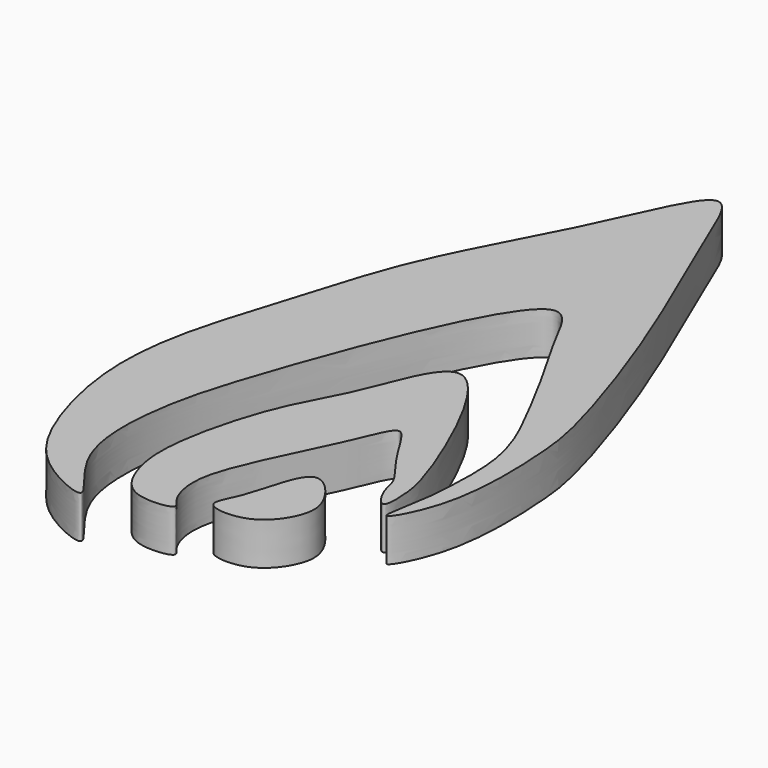
from build123d import *

# Parameters (mm, degrees)
F1_DEPTH = 2
F2_DEPTH = 2
F3_DEPTH = 2
F4_DEPTH = 2


with BuildPart() as f1:
    # F0 (on Top) → F1 (new body)
    with BuildSketch(Plane.XY):
        with BuildLine():
            add(Edge.make_bspline(
                [(-32.5672850013, 3.1219571829), (-32.6859499497, 2.9344991028), (-34.4776351624, 2.7171312474), (-35.5482291656, 4.422494706), (-35.9086575316, 6.979267601), (-34.611998845, 11.8924331283), (-32.9569330674, 14.2587003089), (-31.0572529363, 20.5478369876), (-27.3295341139, 12.1424031349), (-26.9229726713, 10.7124071637), (-26.5708728017, 9.7176922693), (-26.472461483, 7.4433293508), (-27.4288898522, 8.9357533576), (-27.4316160751, 9.7586806997), (-28.5586635899, 11.0276756824), (-29.43657262, 12.6500562765), (-30.0319146302, 13.212745305), (-30.6947550928, 11.4252439161), (-31.545022308, 9.7281548628), (-32.4993893892, 7.6848290523), (-33.4657349014, 5.300914359), (-32.9837784569, 3.6009345385), (-32.5002347384, 3.2278782127), (-32.5672850013, 3.1219571829)],
                knots=[0, 0, 0, 0, 0.0427598375, 0.0885114612, 0.1429678521, 0.2174245524, 0.2812052658, 0.3463628651, 0.4334811223, 0.4785659728, 0.5144888364, 0.5558508718, 0.5893888504, 0.6217535859, 0.6653521731, 0.7125781388, 0.735605816, 0.7774424684, 0.8263525402, 0.8774717718, 0.9318426855, 0.9758390461, 1, 1, 1, 1], degree=3))
        make_face()
    extrude(amount=F1_DEPTH)


with BuildPart() as f1b:
    # F0 (on Top) → F1, piece 2 (new body)
    with BuildSketch(Plane.XY):
        with BuildLine():
            add(Edge.make_bspline(
                [(-31.1676040292, 5.4323091172), (-30.7993501606, 6.418684188), (-30.3741980094, 9.2274078665), (-28.3354307618, 6.8800176439), (-28.3617768024, 5.4459638595), (-29.6176129126, 3.739543043), (-32.0673406587, 3.9210301418), (-31.4167942485, 4.7648483213), (-31.1676040292, 5.4323091172)],
                knots=[0, 0, 0, 0, 0.211357265, 0.3784923335, 0.5268801919, 0.6989923037, 0.856978656, 1, 1, 1, 1], degree=3))
        make_face()
    extrude(amount=F1_DEPTH)


with BuildPart() as f1c:
    # F0 (on Top) → F1, piece 3 (new body)
    with BuildSketch(Plane.XY):
        with BuildLine():
            add(Edge.make_bspline(
                [(-32.1894288063, 34.5448069274), (-32.825469935, 34.4762125634), (-34.5504049583, 29.9655867811), (-37.9764946854, 24.193386846), (-39.4232905162, 18.9333147872), (-41.0370975899, 14.1694669242), (-41.427625747, 9.9543258562), (-40.3540156984, 5.6066084298), (-38.6545034629, 2.7413908895), (-34.8397503257, 1.1295665839), (-38.0567652219, 4.1247207849), (-38.050479764, 8.5944042105), (-36.9532282396, 12.978063641), (-31.8804744587, 26.2758532052), (-29.9546055528, 22.1557119647), (-28.4764532349, 19.6995079994), (-27.0888871093, 17.0538055169), (-25.5830445297, 14.0798259249), (-25.6196484308, 11.0025411486), (-25.7654452938, 9.1099063647), (-26.3325035045, 6.5646973327), (-24.4668055494, 9.8000848112), (-24.6729202706, 14.8589482464), (-24.9750569559, 17.2994506188), (-27.3189450681, 24.5338351747), (-30.5176445119, 31.5190748632), (-31.6920335701, 34.5984489144), (-32.1894288063, 34.5448069274)],
                knots=[0, 0, 0, 0, 0.0422205135, 0.0963935575, 0.1426974097, 0.1868727849, 0.227657643, 0.2690749269, 0.3068969517, 0.3372872054, 0.3691935607, 0.410207351, 0.4574179786, 0.5248366928, 0.5538673244, 0.5892803691, 0.6235760694, 0.6597842759, 0.6939843622, 0.7234180222, 0.747221353, 0.7772543294, 0.8230197464, 0.8546303011, 0.9086196247, 0.9669828234, 1, 1, 1, 1], degree=3))
        make_face()
    extrude(amount=F1_DEPTH)


with BuildPart() as f2:
    # F0 (on Top) → F2 (new body)
    with BuildSketch(Plane.XY):
        with BuildLine():
            add(Edge.make_bspline(
                [(-32.5672850013, 3.1219571829), (-32.6859499497, 2.9344991028), (-34.4776351624, 2.7171312474), (-35.5482291656, 4.422494706), (-35.9086575316, 6.979267601), (-34.611998845, 11.8924331283), (-32.9569330674, 14.2587003089), (-31.0572529363, 20.5478369876), (-27.3295341139, 12.1424031349), (-26.9229726713, 10.7124071637), (-26.5708728017, 9.7176922693), (-26.472461483, 7.4433293508), (-27.4288898522, 8.9357533576), (-27.4316160751, 9.7586806997), (-28.5586635899, 11.0276756824), (-29.43657262, 12.6500562765), (-30.0319146302, 13.212745305), (-30.6947550928, 11.4252439161), (-31.545022308, 9.7281548628), (-32.4993893892, 7.6848290523), (-33.4657349014, 5.300914359), (-32.9837784569, 3.6009345385), (-32.5002347384, 3.2278782127), (-32.5672850013, 3.1219571829)],
                knots=[0, 0, 0, 0, 0.0427598375, 0.0885114612, 0.1429678521, 0.2174245524, 0.2812052658, 0.3463628651, 0.4334811223, 0.4785659728, 0.5144888364, 0.5558508718, 0.5893888504, 0.6217535859, 0.6653521731, 0.7125781388, 0.735605816, 0.7774424684, 0.8263525402, 0.8774717718, 0.9318426855, 0.9758390461, 1, 1, 1, 1], degree=3))
        make_face()
    extrude(amount=F2_DEPTH)


with BuildPart() as f2b:
    # F0 (on Top) → F2, piece 2 (new body)
    with BuildSketch(Plane.XY):
        with BuildLine():
            add(Edge.make_bspline(
                [(-31.1676040292, 5.4323091172), (-30.7993501606, 6.418684188), (-30.3741980094, 9.2274078665), (-28.3354307618, 6.8800176439), (-28.3617768024, 5.4459638595), (-29.6176129126, 3.739543043), (-32.0673406587, 3.9210301418), (-31.4167942485, 4.7648483213), (-31.1676040292, 5.4323091172)],
                knots=[0, 0, 0, 0, 0.211357265, 0.3784923335, 0.5268801919, 0.6989923037, 0.856978656, 1, 1, 1, 1], degree=3))
        make_face()
    extrude(amount=F2_DEPTH)


with BuildPart() as f2c:
    # F0 (on Top) → F2, piece 3 (new body)
    with BuildSketch(Plane.XY):
        with BuildLine():
            add(Edge.make_bspline(
                [(-32.1894288063, 34.5448069274), (-32.825469935, 34.4762125634), (-34.5504049583, 29.9655867811), (-37.9764946854, 24.193386846), (-39.4232905162, 18.9333147872), (-41.0370975899, 14.1694669242), (-41.427625747, 9.9543258562), (-40.3540156984, 5.6066084298), (-38.6545034629, 2.7413908895), (-34.8397503257, 1.1295665839), (-38.0567652219, 4.1247207849), (-38.050479764, 8.5944042105), (-36.9532282396, 12.978063641), (-31.8804744587, 26.2758532052), (-29.9546055528, 22.1557119647), (-28.4764532349, 19.6995079994), (-27.0888871093, 17.0538055169), (-25.5830445297, 14.0798259249), (-25.6196484308, 11.0025411486), (-25.7654452938, 9.1099063647), (-26.3325035045, 6.5646973327), (-24.4668055494, 9.8000848112), (-24.6729202706, 14.8589482464), (-24.9750569559, 17.2994506188), (-27.3189450681, 24.5338351747), (-30.5176445119, 31.5190748632), (-31.6920335701, 34.5984489144), (-32.1894288063, 34.5448069274)],
                knots=[0, 0, 0, 0, 0.0422205135, 0.0963935575, 0.1426974097, 0.1868727849, 0.227657643, 0.2690749269, 0.3068969517, 0.3372872054, 0.3691935607, 0.410207351, 0.4574179786, 0.5248366928, 0.5538673244, 0.5892803691, 0.6235760694, 0.6597842759, 0.6939843622, 0.7234180222, 0.747221353, 0.7772543294, 0.8230197464, 0.8546303011, 0.9086196247, 0.9669828234, 1, 1, 1, 1], degree=3))
        make_face()
    extrude(amount=F2_DEPTH)


with BuildPart() as f3:
    # F0 (on Top) → F3 (new body)
    with BuildSketch(Plane.XY):
        with BuildLine():
            add(Edge.make_bspline(
                [(-32.5672850013, 3.1219571829), (-32.6859499497, 2.9344991028), (-34.4776351624, 2.7171312474), (-35.5482291656, 4.422494706), (-35.9086575316, 6.979267601), (-34.611998845, 11.8924331283), (-32.9569330674, 14.2587003089), (-31.0572529363, 20.5478369876), (-27.3295341139, 12.1424031349), (-26.9229726713, 10.7124071637), (-26.5708728017, 9.7176922693), (-26.472461483, 7.4433293508), (-27.4288898522, 8.9357533576), (-27.4316160751, 9.7586806997), (-28.5586635899, 11.0276756824), (-29.43657262, 12.6500562765), (-30.0319146302, 13.212745305), (-30.6947550928, 11.4252439161), (-31.545022308, 9.7281548628), (-32.4993893892, 7.6848290523), (-33.4657349014, 5.300914359), (-32.9837784569, 3.6009345385), (-32.5002347384, 3.2278782127), (-32.5672850013, 3.1219571829)],
                knots=[0, 0, 0, 0, 0.0427598375, 0.0885114612, 0.1429678521, 0.2174245524, 0.2812052658, 0.3463628651, 0.4334811223, 0.4785659728, 0.5144888364, 0.5558508718, 0.5893888504, 0.6217535859, 0.6653521731, 0.7125781388, 0.735605816, 0.7774424684, 0.8263525402, 0.8774717718, 0.9318426855, 0.9758390461, 1, 1, 1, 1], degree=3))
        make_face()
    extrude(amount=F3_DEPTH)


with BuildPart() as f3b:
    # F0 (on Top) → F3, piece 2 (new body)
    with BuildSketch(Plane.XY):
        with BuildLine():
            add(Edge.make_bspline(
                [(-31.1676040292, 5.4323091172), (-30.7993501606, 6.418684188), (-30.3741980094, 9.2274078665), (-28.3354307618, 6.8800176439), (-28.3617768024, 5.4459638595), (-29.6176129126, 3.739543043), (-32.0673406587, 3.9210301418), (-31.4167942485, 4.7648483213), (-31.1676040292, 5.4323091172)],
                knots=[0, 0, 0, 0, 0.211357265, 0.3784923335, 0.5268801919, 0.6989923037, 0.856978656, 1, 1, 1, 1], degree=3))
        make_face()
    extrude(amount=F3_DEPTH)


with BuildPart() as f3c:
    # F0 (on Top) → F3, piece 3 (new body)
    with BuildSketch(Plane.XY):
        with BuildLine():
            add(Edge.make_bspline(
                [(-32.1894288063, 34.5448069274), (-32.825469935, 34.4762125634), (-34.5504049583, 29.9655867811), (-37.9764946854, 24.193386846), (-39.4232905162, 18.9333147872), (-41.0370975899, 14.1694669242), (-41.427625747, 9.9543258562), (-40.3540156984, 5.6066084298), (-38.6545034629, 2.7413908895), (-34.8397503257, 1.1295665839), (-38.0567652219, 4.1247207849), (-38.050479764, 8.5944042105), (-36.9532282396, 12.978063641), (-31.8804744587, 26.2758532052), (-29.9546055528, 22.1557119647), (-28.4764532349, 19.6995079994), (-27.0888871093, 17.0538055169), (-25.5830445297, 14.0798259249), (-25.6196484308, 11.0025411486), (-25.7654452938, 9.1099063647), (-26.3325035045, 6.5646973327), (-24.4668055494, 9.8000848112), (-24.6729202706, 14.8589482464), (-24.9750569559, 17.2994506188), (-27.3189450681, 24.5338351747), (-30.5176445119, 31.5190748632), (-31.6920335701, 34.5984489144), (-32.1894288063, 34.5448069274)],
                knots=[0, 0, 0, 0, 0.0422205135, 0.0963935575, 0.1426974097, 0.1868727849, 0.227657643, 0.2690749269, 0.3068969517, 0.3372872054, 0.3691935607, 0.410207351, 0.4574179786, 0.5248366928, 0.5538673244, 0.5892803691, 0.6235760694, 0.6597842759, 0.6939843622, 0.7234180222, 0.747221353, 0.7772543294, 0.8230197464, 0.8546303011, 0.9086196247, 0.9669828234, 1, 1, 1, 1], degree=3))
        make_face()
    extrude(amount=F3_DEPTH)


with BuildPart() as f4:
    # F0 (on Top) → F4 (new body)
    with BuildSketch(Plane.XY):
        with BuildLine():
            add(Edge.make_bspline(
                [(-32.5672850013, 3.1219571829), (-32.6859499497, 2.9344991028), (-34.4776351624, 2.7171312474), (-35.5482291656, 4.422494706), (-35.9086575316, 6.979267601), (-34.611998845, 11.8924331283), (-32.9569330674, 14.2587003089), (-31.0572529363, 20.5478369876), (-27.3295341139, 12.1424031349), (-26.9229726713, 10.7124071637), (-26.5708728017, 9.7176922693), (-26.472461483, 7.4433293508), (-27.4288898522, 8.9357533576), (-27.4316160751, 9.7586806997), (-28.5586635899, 11.0276756824), (-29.43657262, 12.6500562765), (-30.0319146302, 13.212745305), (-30.6947550928, 11.4252439161), (-31.545022308, 9.7281548628), (-32.4993893892, 7.6848290523), (-33.4657349014, 5.300914359), (-32.9837784569, 3.6009345385), (-32.5002347384, 3.2278782127), (-32.5672850013, 3.1219571829)],
                knots=[0, 0, 0, 0, 0.0427598375, 0.0885114612, 0.1429678521, 0.2174245524, 0.2812052658, 0.3463628651, 0.4334811223, 0.4785659728, 0.5144888364, 0.5558508718, 0.5893888504, 0.6217535859, 0.6653521731, 0.7125781388, 0.735605816, 0.7774424684, 0.8263525402, 0.8774717718, 0.9318426855, 0.9758390461, 1, 1, 1, 1], degree=3))
        make_face()
    extrude(amount=F4_DEPTH)


with BuildPart() as f4b:
    # F0 (on Top) → F4, piece 2 (new body)
    with BuildSketch(Plane.XY):
        with BuildLine():
            add(Edge.make_bspline(
                [(-31.1676040292, 5.4323091172), (-30.7993501606, 6.418684188), (-30.3741980094, 9.2274078665), (-28.3354307618, 6.8800176439), (-28.3617768024, 5.4459638595), (-29.6176129126, 3.739543043), (-32.0673406587, 3.9210301418), (-31.4167942485, 4.7648483213), (-31.1676040292, 5.4323091172)],
                knots=[0, 0, 0, 0, 0.211357265, 0.3784923335, 0.5268801919, 0.6989923037, 0.856978656, 1, 1, 1, 1], degree=3))
        make_face()
    extrude(amount=F4_DEPTH)


with BuildPart() as f4c:
    # F0 (on Top) → F4, piece 3 (new body)
    with BuildSketch(Plane.XY):
        with BuildLine():
            add(Edge.make_bspline(
                [(-32.1894288063, 34.5448069274), (-32.825469935, 34.4762125634), (-34.5504049583, 29.9655867811), (-37.9764946854, 24.193386846), (-39.4232905162, 18.9333147872), (-41.0370975899, 14.1694669242), (-41.427625747, 9.9543258562), (-40.3540156984, 5.6066084298), (-38.6545034629, 2.7413908895), (-34.8397503257, 1.1295665839), (-38.0567652219, 4.1247207849), (-38.050479764, 8.5944042105), (-36.9532282396, 12.978063641), (-31.8804744587, 26.2758532052), (-29.9546055528, 22.1557119647), (-28.4764532349, 19.6995079994), (-27.0888871093, 17.0538055169), (-25.5830445297, 14.0798259249), (-25.6196484308, 11.0025411486), (-25.7654452938, 9.1099063647), (-26.3325035045, 6.5646973327), (-24.4668055494, 9.8000848112), (-24.6729202706, 14.8589482464), (-24.9750569559, 17.2994506188), (-27.3189450681, 24.5338351747), (-30.5176445119, 31.5190748632), (-31.6920335701, 34.5984489144), (-32.1894288063, 34.5448069274)],
                knots=[0, 0, 0, 0, 0.0422205135, 0.0963935575, 0.1426974097, 0.1868727849, 0.227657643, 0.2690749269, 0.3068969517, 0.3372872054, 0.3691935607, 0.410207351, 0.4574179786, 0.5248366928, 0.5538673244, 0.5892803691, 0.6235760694, 0.6597842759, 0.6939843622, 0.7234180222, 0.747221353, 0.7772543294, 0.8230197464, 0.8546303011, 0.9086196247, 0.9669828234, 1, 1, 1, 1], degree=3))
        make_face()
    extrude(amount=F4_DEPTH)


solid = Compound([f1.part, f1b.part, f1c.part, f2.part, f2b.part, f2c.part, f3.part, f3b.part, f3c.part, f4.part, f4b.part, f4c.part])
